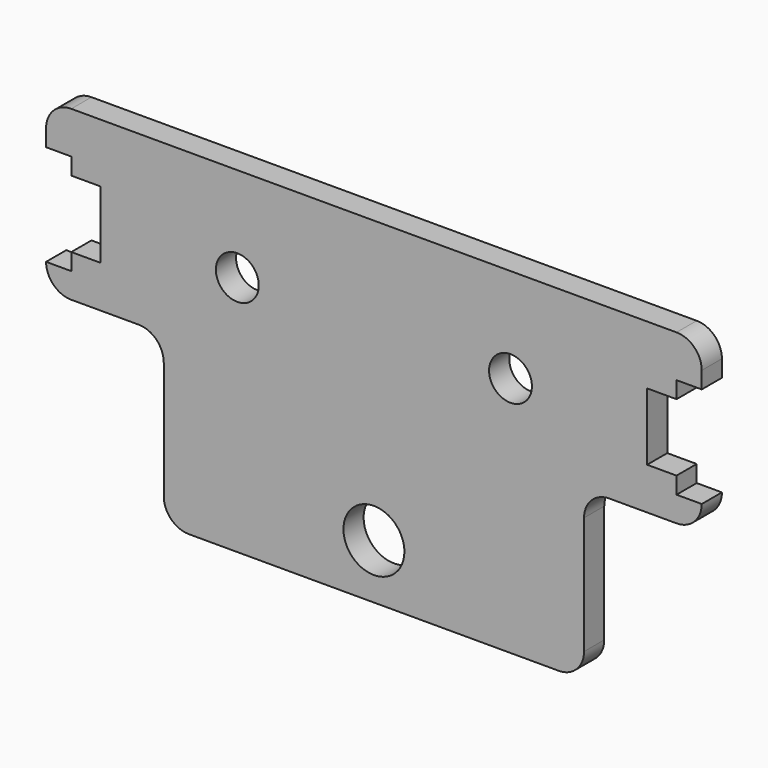
from build123d import *
from build123d import SkipClean  # not in build123d's __all__

# Parameters (mm, degrees)
F1_DEPTH = 6
F2_R     = 5.1
F3_DEPTH = 25
F5_DEPTH = 25
F6_R     = 5.99999
F8_R     = 6


# Not quite as in the source:
# - a fillet or chamfer is up to 0.001 mm smaller than in the source, because OpenCascade refuses the exact size


with BuildPart() as f1:
    # F0 (on Front) → F1 (new body)
    with BuildSketch(Plane.XZ):
        Polygon((-50, 0), (0, 0), (0, 80), (-78, 80), (-78, 70), (-72, 70), (-72, 66), (-65, 66), (-65, 50), (-72, 50), (-72, 46), (-78, 46), (-78, 40), (-50, 40), align=None)
    extrude(amount=F1_DEPTH)

    # F2 (on face) → F3 (cut)
    with BuildSketch(Plane.XZ.offset(6)):
        with Locations((-32.5, 57.5)):
            Circle(F2_R)
    extrude(amount=-F3_DEPTH, mode=Mode.SUBTRACT)

    # F4 (on face) → F5 (cut)
    with BuildSketch(Plane.XZ.offset(6)):
        with BuildLine():
            Line((0, 5.75), (0, 20.25))
            ThreePointArc((0, 20.25), (-7.25, 13), (0, 5.75))
        make_face()
    extrude(amount=-F5_DEPTH, mode=Mode.SUBTRACT)

    # F6 (radius 6 in the source; OpenCascade refuses exactly that, so slightly less here)
    f6_edges = [f1.edges().sort_by_distance(p)[0] for p in [
        (-78, -3, 80),
        (-78, -3, 40),
        (-50, -3, 0),
    ]]
    fillet(f6_edges, radius=F6_R)

    # F7: F1 across face


with BuildPart() as f1_1:
    add(f1.part, clean=False)
    with SkipClean():  # cleaning this boolean's faces spoils the solid; the shape is the same uncleaned
        add(f1.part.mirror(Plane(origin=(0, -3, 50.125), x_dir=(0, 1, 0), z_dir=(1, 0, 0))), clean=False)

    # F8
    f8_edges = [f1_1.edges().sort_by_distance(p)[0] for p in [
        (-50, -3, 40),
        (50, -3, 40),
    ]]
    fillet(f8_edges, radius=F8_R)


solid = f1_1.part
